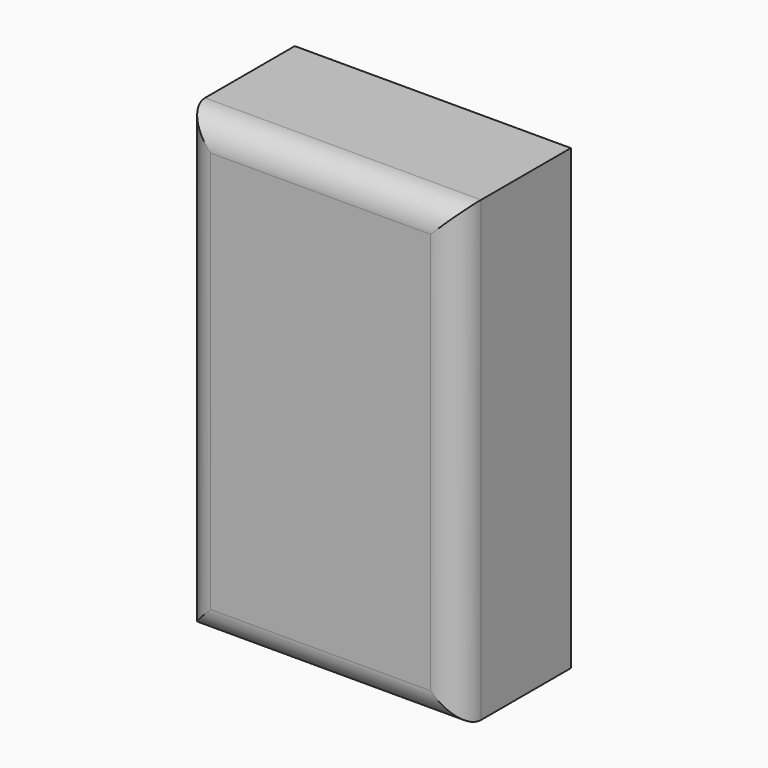
from build123d import *

# Parameters (mm, degrees)
F0_W     = 50.0062517822
F0_H     = 82.9441100359
F1_DEPTH = 25.4
F2_R     = 5.08
F3_T     = -2.54


# Not quite as in the source:
# - the program builds the solid bodies; features that only make, move or delete a surface that nothing else refers to are left out


with BuildPart() as f1:
    # F0 (on Front) → F1 (new body)
    with BuildSketch(Plane.XZ):
        with Locations((47.5059393793, 78.971914947)):
            Rectangle(F0_W, F0_H)
    extrude(amount=F1_DEPTH)

    # F2
    f2_edges = [f1.edges().sort_by_distance(p)[0] for p in [
        (72.509065, -25.4, 78.971915),
        (22.502813, -25.4, 78.971915),
        (47.505939, -25.4, 120.44397),
        (47.505939, -25.4, 37.49986),
    ]]
    fillet(f2_edges, radius=F2_R)

    # F3
    f3_openings = [f1.faces().sort_by_distance(p)[0] for p in [
        (47.505939, 0, 78.971915),
    ]]
    offset(amount=F3_T, openings=f3_openings)


solid = f1.part
